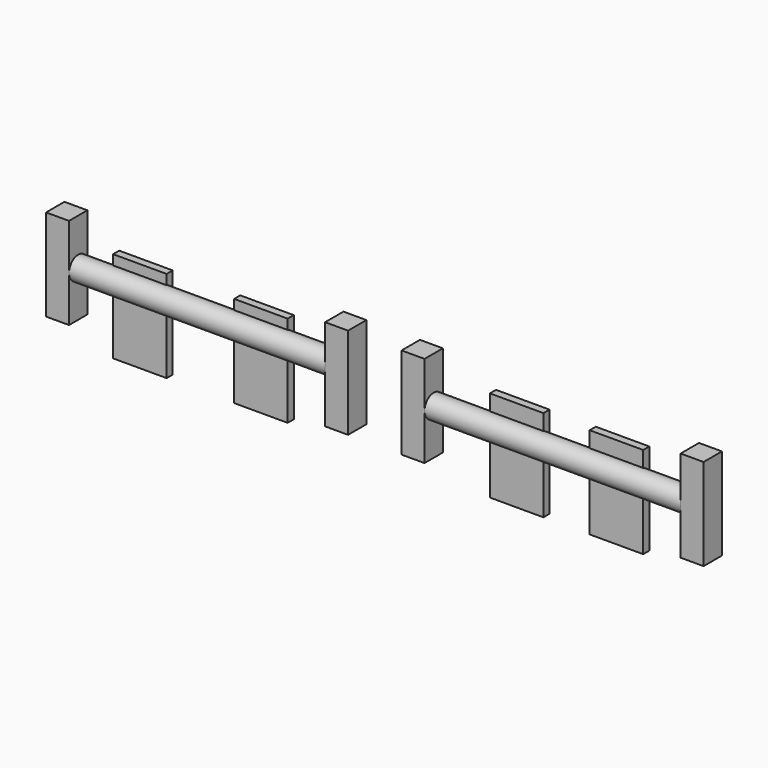
from build123d import *

# Parameters (mm, degrees)
F0_W     = 38.1
F0_H     = 152.4
F1_DEPTH = 38.1
F3_DEPTH = 457.2
F4_R     = 19.05
F5_DEPTH = 457.2
F6_W     = 88.9
F6_H     = 152.4
F7_DEPTH = 12.7


with BuildPart() as f1:
    # F0 (on Front) → F1 (new body)
    with BuildSketch(Plane.XZ):
        with Locations((-182.7645437746, -34.3906155205)):
            Rectangle(F0_W, F0_H)
    extrude(amount=F1_DEPTH)

    # F2 (on face) → F3 (join)
    with BuildSketch(Plane.YZ.offset(-163.7145437746)):
        with BuildLine():
            ThreePointArc((-38.1, -34.3906155205), (-19.05, -53.4406155205), (0, -34.3906155205))
            ThreePointArc((0, -34.3906155205), (-19.05, -15.3406155205), (-38.1, -34.3906155205))
        make_face()
    extrude(amount=F3_DEPTH)


with BuildPart() as f1b:
    # F0 (on Front) → F1, piece 2 (new body)
    with BuildSketch(Plane.XZ):
        with Locations((280.7854562254, -44.1833949373)):
            Rectangle(F0_W, F0_H)
    extrude(amount=F1_DEPTH)


with BuildPart() as f1c:
    # F0 (on Front) → F1, piece 3 (new body)
    with BuildSketch(Plane.XZ):
        with Locations((407.7854562254, -44.1833949373)):
            Rectangle(F0_W, F0_H)
    extrude(amount=F1_DEPTH)


with BuildPart() as f1d:
    # F0 (on Front) → F1, piece 4 (new body)
    with BuildSketch(Plane.XZ):
        with Locations((871.3354562254, -44.1833949373)):
            Rectangle(F0_W, F0_H)
    extrude(amount=F1_DEPTH)


with BuildPart() as f5:
    # F4 (on face) → F5 (new body)
    with BuildSketch(Plane(origin=(852.2854562254, 0, 0), x_dir=(0, -1, 0), z_dir=(-1, 0, 0))):
        with Locations((19.05, -44.1833949373)):
            Circle(F4_R)
    extrude(amount=F5_DEPTH)


with BuildPart() as f7:
    # F6 (on Front) → F7 (new body)
    with BuildSketch(Plane.XZ):
        with Locations((134.7354562254, -76.2)):
            Rectangle(F6_W, F6_H)
    extrude(amount=F7_DEPTH)


with BuildPart() as f7b:
    # F6 (on Front) → F7, piece 2 (new body)
    with BuildSketch(Plane.XZ):
        with Locations((725.2854562254, -76.2)):
            Rectangle(F6_W, F6_H)
    extrude(amount=F7_DEPTH)


with BuildPart() as f7c:
    # F6 (on Front) → F7, piece 3 (new body)
    with BuildSketch(Plane.XZ):
        with Locations((559.5377833366, -76.2)):
            Rectangle(F6_W, F6_H)
    extrude(amount=F7_DEPTH)


with BuildPart() as f7d:
    # F6 (on Front) → F7, piece 4 (new body)
    with BuildSketch(Plane.XZ):
        with Locations((-66.3621499419, -76.2)):
            Rectangle(F6_W, F6_H)
    extrude(amount=F7_DEPTH)


solid = Compound([f1.part, f1b.part, f1c.part, f1d.part, f5.part, f7.part, f7b.part, f7c.part, f7d.part])
